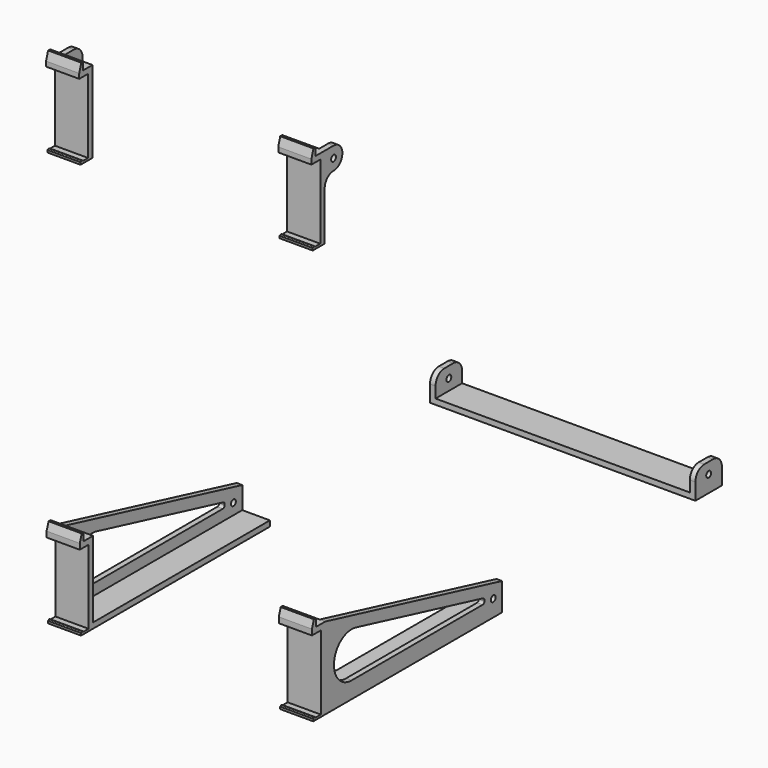
from build123d import *

# Parameters (mm, degrees)
F1_DEPTH  = 30
F2_R      = 2.75
F3_DEPTH  = 5
F4_R      = 20
F5_R      = 2
F7_DEPTH  = 30
F8_W      = 20
F8_H      = 20
F8_R      = 2.75
F9_DEPTH  = 5
F10_R     = 9.99999
F11_R     = 2.75
F12_DEPTH = 5
F13_R     = 10
F14_W     = 115
F14_H     = 5
F15_DEPTH = 30


# Not quite as in the source:
# - a fillet or chamfer is up to 0.001 mm smaller than in the source, because OpenCascade refuses the exact size


with BuildPart() as f1:
    # F0 (on Right) → F1 (new body)
    with BuildSketch(Plane.YZ):
        Polygon((2.6676042763, 31.7598315338), (2.6676042763, -35.2401684662), (-2.8323957237, -35.2401684662), (-4.3323957237, -34.4901684662), (-5.8323957237, -35.2401684662), (-5.8323957237, -37.2401684662), (7.6676042763, -37.2401684662), (207.6676042763, -37.2401684662), (207.6676042763, -32.2401684662), (7.6676042763, -32.2401684662), (7.6676042763, 36.7598315338), (-2.8323957237, 36.7598315338), (-2.8323957237, 43.7598315338), (-5.0823957237, 43.7598315338), (-7.3323957237, 36.874037236), (-7.3323957237, 31.7598315338), align=None)
    extrude(amount=F1_DEPTH)

    # F2 (on face) → F3 (join)
    with BuildSketch(Plane.YZ.offset(30)):
        Polygon((207.6676042763, -12.2401684662), (7.6676042763, 36.7598315338), (7.6676042763, -32.2401684662), (207.6676042763, -32.2401684662), align=None)
        with Locations((197.6676042763, -22.2401684662)):
            Circle(F2_R, mode=Mode.SUBTRACT)
        Polygon((187.6676042763, -17.6359200172), (187.6676042763, -22.2401684662), (17.6676042763, -22.2401684662), (17.6676042763, 24.0140799828), align=None, mode=Mode.SUBTRACT)
    extrude(amount=-F3_DEPTH)

    # F4
    f4_edges = [f1.edges().sort_by_distance(p)[0] for p in [
        (27.5, 17.667604, -22.240168),
        (27.5, 17.667604, 24.01408),
    ]]
    fillet(f4_edges, radius=F4_R)

    # F5
    f5_edges = [f1.edges().sort_by_distance(p)[0] for p in [
        (27.5, 187.667604, -22.240168),
        (27.5, 187.667604, -17.63592),
    ]]
    fillet(f5_edges, radius=F5_R)


with BuildPart() as f7:
    # F6 (on Right) → F7 (new body)
    with BuildSketch(Plane.YZ):
        Polygon((2.0973396314, 406.8939414024), (2.0973396314, 339.8939414024), (-3.4026603686, 339.8939414024), (-4.9026603686, 340.6439414024), (-6.4026603686, 339.8939414024), (-6.4026603686, 337.8939414024), (7.0973396314, 337.8939414024), (7.0973396314, 411.8939414024), (-3.4026603686, 411.8939414024), (-3.4026603686, 418.8939414024), (-5.6526603686, 418.8939414024), (-7.9026603686, 411.3168716431), (-7.9026603686, 406.8939414024), align=None)
    extrude(amount=F7_DEPTH)

    # F8 (on face) → F9 (join)
    with BuildSketch(Plane.YZ.offset(30)):
        with Locations((17.0973396314, 401.8939414024)):
            Rectangle(F8_W, F8_H)
        with Locations((17.0973396314, 401.8939414024)):
            Circle(F8_R, mode=Mode.SUBTRACT)
    extrude(amount=-F9_DEPTH)

    # F10 (radius 10 in the source; OpenCascade refuses exactly that, so slightly less here)
    f10_edges = [f7.edges().sort_by_distance(p)[0] for p in [
        (27.5, 27.09734, 411.893941),
        (27.5, 27.09734, 391.893941),
        (27.5, 7.09734, 391.893941),
    ]]
    fillet(f10_edges, radius=F10_R)


with BuildPart() as f12:
    # F11 (on face) → F12 (new body)
    with BuildSketch(Plane.YZ.offset(30)):
        Polygon((426.2179685545, -37.2266875207), (441.2179685545, -37.2266875207), (456.2179685545, -37.2266875207), (456.2179685545, -12.2266875207), (426.2179685545, -12.2266875207), align=None)
        with Locations((441.2179685545, -22.2266875207)):
            Circle(F11_R, mode=Mode.SUBTRACT)
    extrude(amount=-F12_DEPTH)

    # F13
    f13_edges = [f12.edges().sort_by_distance(p)[0] for p in [
        (27.5, 426.217969, -12.226688),
        (27.5, 456.217969, -12.226688),
    ]]
    fillet(f13_edges, radius=F13_R)

    # F14 (on face) → F15 (join)
    with BuildSketch(Plane(origin=(0, 456.2179685545, 0), x_dir=(-1, 0, 0), z_dir=(0, 1, 0))):
        with Locations((32.5, -34.7266875207)):
            Rectangle(F14_W, F14_H)
    extrude(amount=-F15_DEPTH)

    # F17: F12 across plane


with BuildPart() as f12_1:
    add(f12.part)
    add(f12.part.mirror(Plane.YZ.offset(-90)))


with BuildPart() as f18_1:
    # F18: instance of F1
    add(f1.part.mirror(Plane.YZ.offset(-90)))


with BuildPart() as f18_2:
    # F18: instance of F7
    add(f7.part.mirror(Plane.YZ.offset(-90)))


solid = Compound([f1.part, f7.part, f12_1.part, f18_1.part, f18_2.part])
